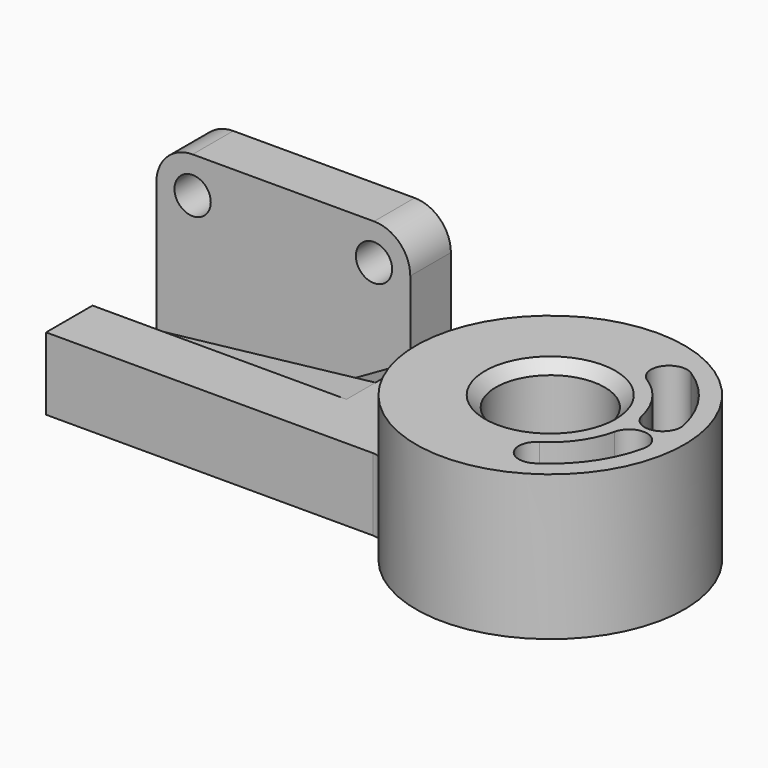
from build123d import *

# Parameters (mm, degrees)
F0_R         = 15
F1_DEPTH     = 40
F2_DEPTH     = 20
F4_DEPTH     = 10
F3_W         = 70
F3_H         = 8
F5_DEPTH     = 12
F6_W         = 70
F6_H         = 14
F7_DEPTH     = 31
F9_DEPTH     = 14.001
F0_W         = 28
F0_H         = 12
F10_DEPTH    = 20
F11_T1_DEPTH = 12
F12_SIZE     = 3


# Not quite as in the source:
# - a fillet or chamfer that OpenCascade refuses, or shapes differently, is made with other operations: its cross-section is extruded or revolved along the edge and cut away or added
# - a feature names something its author has since deleted; it is built from what else it names


with BuildPart() as f1:
    # F0 (on Top) → F1 (new body)
    with BuildSketch(Plane.XY):
        with BuildLine():
            ThreePointArc((18.202077895, 19.380952381), (59.8256579019, 1.1334458447), (87.7377377315, 37))
            ThreePointArc((87.7377377315, 37), (76.9006886354, 63.1629509039), (50.7377377315, 74))
            ThreePointArc((50.7377377315, 74), (18.9501240911, 55.9353536816), (18.202077895, 19.380952381))
        make_face()
        with BuildLine():
            ThreePointArc((81.9861465659, 30.1052958497), (76.9690140278, 18.6718756042), (67.9584074606, 10.028746153))
            ThreePointArc((67.9584074606, 10.028746153), (61.0534194019, 11.5522749214), (62.5769481703, 18.4572629802))
            ThreePointArc((62.5769481703, 18.4572629802), (28.7377377315, 37), (62.5769481703, 55.5427370198))
            ThreePointArc((62.5769481703, 55.5427370198), (61.0534194019, 62.4477250786), (67.9584074606, 63.971253847))
            ThreePointArc((67.9584074606, 63.971253847), (76.9690140278, 55.3281243958), (81.9861465659, 43.8947041503))
            ThreePointArc((81.9861465659, 43.8947041503), (78.180880209, 37.9348427464), (72.2210188051, 41.7401091033))
            ThreePointArc((72.2210188051, 41.7401091033), (72.6081764973, 39.3840948366), (72.7377377315, 37))
            ThreePointArc((72.7377377315, 37), (72.6081764973, 34.6159051634), (72.2210188051, 32.2598908967))
            ThreePointArc((72.2210188051, 32.2598908967), (78.180880209, 36.0651572536), (81.9861465659, 30.1052958497))
        make_face(mode=Mode.SUBTRACT)
        with BuildLine():
            ThreePointArc((62.5769481703, 55.5427370198), (28.7377377315, 37), (62.5769481703, 18.4572629802))
            ThreePointArc((62.5769481703, 18.4572629802), (68.7717401852, 24.3994144779), (72.2210188051, 32.2598908967))
            ThreePointArc((72.2210188051, 32.2598908967), (72.6081764973, 34.6159051634), (72.7377377315, 37))
            ThreePointArc((72.7377377315, 37), (72.6081764973, 39.3840948366), (72.2210188051, 41.7401091033))
            ThreePointArc((72.2210188051, 41.7401091033), (68.7717401852, 49.6005855221), (62.5769481703, 55.5427370198))
        make_face()
        with Locations((50.7377377315, 37)):
            Circle(F0_R, mode=Mode.SUBTRACT)
    extrude(amount=F1_DEPTH)

    # F12
    f12_edges = [f1.edges().sort_by_distance(p)[0] for p in [
        (35.737738, 37, 40),
    ]]
    chamfer(f12_edges, length=F12_SIZE)


with BuildPart() as f2:
    # F0 (on Top) → F2 (new body)
    with BuildSketch(Plane.XY):
        with BuildLine():
            ThreePointArc((18.202077895, 19.380952381), (18.9501240911, 55.9353536816), (50.7377377315, 74))
            Line((50.7377377315, 74), (-6.2622622685, 74))
            Line((-6.2622622685, 74), (-6.2622622685, 60))
            Line((-6.2622622685, 60), (-6.2622622685, 48))
            Line((-6.2622622685, 48), (-6.2622622685, 36))
            Line((-6.2622622685, 36), (-6.2622622685, 22))
            Line((-6.2622622685, 22), (13.8053671063, 22))
            ThreePointArc((13.8053671063, 22), (16.3641986849, 21.2956234649), (18.202077895, 19.380952381))
        make_face()
        Polygon((-12.395917438, 22), (-6.2622622685, 22), (-6.2622622685, 36), (-76.2622622685, 36), (-76.2622622685, 22), align=None)
        Polygon((-6.2622622685, 36), (-6.2622622685, 48), (-34.2622622685, 48), (-76.2622622685, 48), (-76.2622622685, 36), align=None)
        Polygon((-6.2622622685, 60), (-6.2622622685, 74), (-76.2622622685, 74), (-76.2622622685, 60), (-34.2622622685, 60), align=None)
    extrude(amount=F2_DEPTH)

    # F3 (on face) → F4 (cut)
    with BuildSketch(Plane(origin=(0, 48, 0), x_dir=(-1, 0, 0), z_dir=(0, 1, 0))):
        Polygon((76.2622622685, 12), (76.2622622685, 20), (6.2622622685, 20), align=None)
    extrude(amount=-F4_DEPTH, mode=Mode.SUBTRACT)

    # F3 (on face) → F5 (cut)
    with BuildSketch(Plane(origin=(0, 48, 0), x_dir=(-1, 0, 0), z_dir=(0, 1, 0))):
        with Locations((41.2622622685, 4)):
            Rectangle(F3_W, F3_H)
    extrude(amount=-F5_DEPTH, mode=Mode.SUBTRACT)

    # F6 (on face) → F7 (join)
    with BuildSketch(Plane.XY.offset(20)):
        with Locations((-41.2622622685, 67)):
            Rectangle(F6_W, F6_H)
    extrude(amount=F7_DEPTH)

    # F8 (on face) → F9 (cut, through all)
    with BuildSketch(Plane.XZ.offset(-60)):
        with BuildLine():
            ThreePointArc((-61.2622622685, 41), (-62.7267283626, 44.5355339059), (-66.2622622685, 46))
            ThreePointArc((-66.2622622685, 46), (-69.7977961744, 37.4644660941), (-61.2622622685, 41))
        make_face()
        with BuildLine():
            ThreePointArc((-76.2622622685, 41), (-73.3333300804, 48.0710678119), (-66.2622622685, 51))
            Line((-66.2622622685, 51), (-76.2622622685, 51))
            Line((-76.2622622685, 51), (-76.2622622685, 41))
        make_face()
        with BuildLine():
            Line((-6.2622622685, 41), (-6.2622622685, 51))
            Line((-6.2622622685, 51), (-16.2622622685, 51))
            ThreePointArc((-16.2622622685, 51), (-9.1911944566, 48.0710678119), (-6.2622622685, 41))
        make_face()
        with BuildLine():
            ThreePointArc((-11.2622622685, 41), (-12.7267283626, 44.5355339059), (-16.2622622685, 46))
            ThreePointArc((-16.2622622685, 46), (-19.7977961744, 37.4644660941), (-11.2622622685, 41))
        make_face()
    extrude(amount=-F9_DEPTH, mode=Mode.SUBTRACT)

    # F0 (on Top) → F10 (join)
    with BuildSketch(Plane.XY):
        with Locations((-20.2622622685, 54)):
            Rectangle(F0_W, F0_H)
    extrude(amount=F10_DEPTH)

    # F11: chamfer of 28 x 16 on 1 edges, made by hand

    # F11_s2 → F11_t1 (cut)
    with BuildSketch(Plane.XZ.offset(-60)):
        Polygon((-6.2622622685, 20), (-34.2622622685, 4), (-34.2622622685, 20), align=None)
    extrude(amount=F11_T1_DEPTH, mode=Mode.SUBTRACT)


solid = Compound([f1.part, f2.part])
